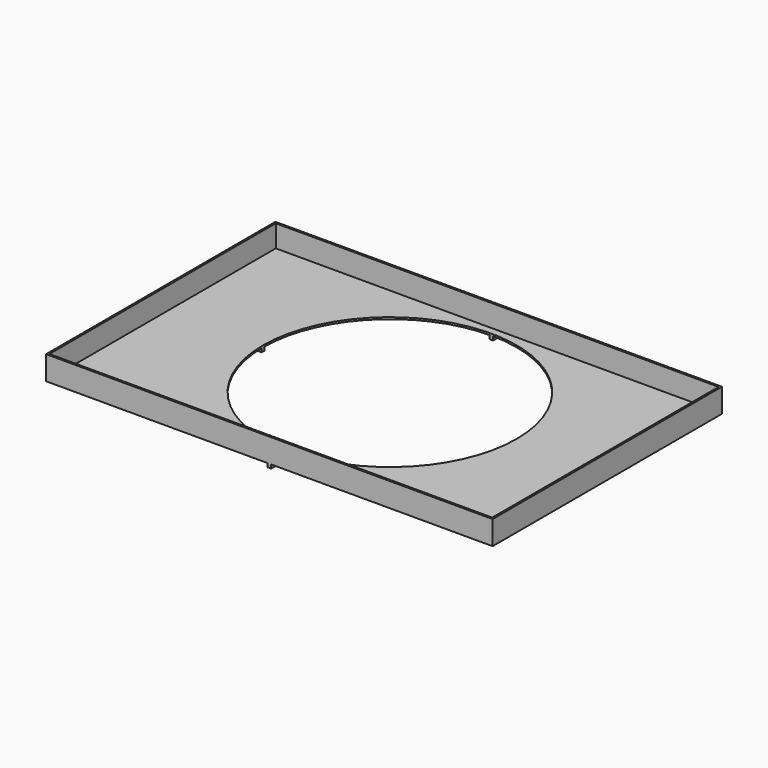
from build123d import *

# Parameters (mm, degrees)
F0_W          = 121.5
F0_H          = 78
F1_DEPTH      = 0.5
F2_W          = 121.5
F2_H          = 78
F2_W_2        = 120.5
F2_H_2        = 77
F3_DEPTH      = 6
F4_R          = 34.5
F5_DEPTH      = 0.501
F6_W          = 1
F6_H          = 6.5
F7_DEPTH      = 1
F8_W          = 1
F8_H          = 2.5
F9_DEPTH      = 1
F10_W         = 6
F10_H         = 1
F11_DEPTH     = 1
F12_W         = 6
F12_H         = 1
F13_DEPTH     = 1
F16_TEXT_SIZE = 7.6388888889
F17_DEPTH     = 1


# Not quite as in the source:
# - Text() gives the source's letters only with a copy of the font that has no kerning and outlines rounded to 1/6400 em; it was checked with that copy


with BuildPart() as f1:
    # F0 (on Top) → F1 (new body)
    with BuildSketch(Plane.XY):
        with Locations((0, -2)):
            Rectangle(F0_W, F0_H)
    extrude(amount=F1_DEPTH)

    # F2 (on face) → F3 (join)
    with BuildSketch(Plane.XY.offset(0.5)):
        with Locations((0, -2)):
            Rectangle(F2_W, F2_H)
        with Locations((0, -2)):
            Rectangle(F2_W_2, F2_H_2, mode=Mode.SUBTRACT)
    extrude(amount=F3_DEPTH)

    # F4 (on face) → F5 (cut, through all)
    with BuildSketch(Plane.XY.offset(0.5)):
        Circle(F4_R)
    extrude(amount=-F5_DEPTH, mode=Mode.SUBTRACT)

    # F6 (on face) → F7 (join)
    with BuildSketch(Plane.XY):
        with Locations((0, -37.75)):
            Rectangle(F6_W, F6_H)
    extrude(amount=-F7_DEPTH)

    # F8 (on face) → F9 (join)
    with BuildSketch(Plane.XY):
        with Locations((0, 35.75)):
            Rectangle(F8_W, F8_H)
    extrude(amount=-F9_DEPTH)

    # F10 (on face) → F11 (join)
    with BuildSketch(Plane.XY):
        with Locations((37.5, 0)):
            Rectangle(F10_W, F10_H)
    extrude(amount=-F11_DEPTH)

    # F12 (on face) → F13 (join)
    with BuildSketch(Plane.XY):
        with Locations((-37.5, 0)):
            Rectangle(F12_W, F12_H)
    extrude(amount=-F13_DEPTH)

    # F16 (on line) → F17 (join)
    with BuildSketch(Plane(origin=(0, 0, 0), x_dir=(1, 0, 0), z_dir=(0, 0, -1))):
        with Locations((-59.25, -2.75)):
            Text('West', F16_TEXT_SIZE, font='Open Sans', text_align=(TextAlign.LEFT, TextAlign.BOTTOM))
        with Locations((41.0784505208, -2.75)):
            Text('East', F16_TEXT_SIZE, font='Open Sans', text_align=(TextAlign.LEFT, TextAlign.BOTTOM))
    extrude(amount=F17_DEPTH)


solid = f1.part
